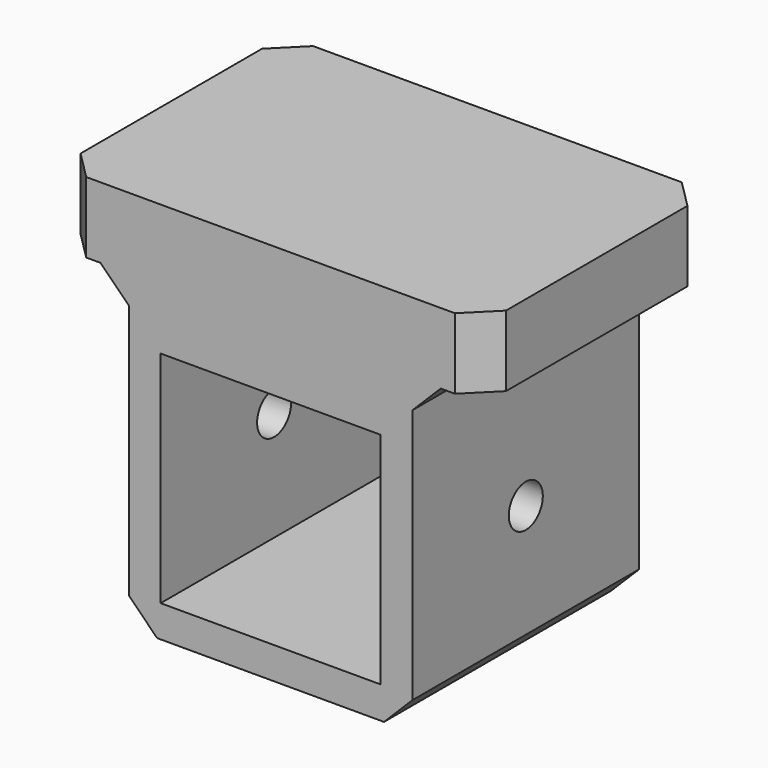
from build123d import *

# Parameters (mm, degrees)
F0_W          = 20
F0_H          = 22
F0_W_2        = 15.5
F0_H_2        = 15.5
F1_DEPTH      = 20
F2_SIZE       = 2
F3_R          = 1.5
F4_DEPTH      = 7.251
F4_DEPTH_BACK = 25


# Not quite as in the source:
# - a feature names something its author has since deleted; it is built from what else it names


with BuildPart() as f1:
    # F0 (on Front) → F1 (new body)
    with BuildSketch(Plane.XZ):
        with Locations((-38.0418774337, 18.7455339581)):
            Rectangle(F0_W, F0_H)
        with Locations((-38.0418774337, 17.7455339581)):
            Rectangle(F0_W_2, F0_H_2, mode=Mode.SUBTRACT)
        Polygon((-48.0418774337, 29.7455339581), (-28.0418774337, 29.7455339581), (-23.0418774337, 29.7455339581), (-23.0418774337, 34.7455339581), (-53.0418774337, 34.7455339581), (-53.0418774337, 29.7455339581), align=None)
    extrude(amount=F1_DEPTH)

    # F2
    f2_edges = [f1.edges().sort_by_distance(p)[0] for p in [
        (-28.041877, -10, 7.745534),
        (-48.041877, -10, 7.745534),
        (-48.041877, -10, 29.745534),
        (-28.041877, -10, 29.745534),
        (-23.041877, 0, 32.245534),
        (-53.041877, 0, 32.245534),
        (-53.041877, -20, 32.245534),
        (-23.041877, -20, 32.245534),
    ]]
    chamfer(f2_edges, length=F2_SIZE)

    # F3 (on face) → F4 (cut, two sides)
    with BuildSketch(Plane.YZ.offset(-45.7918774337)) as f4_sk:
        with Locations((-10, 17.7455339581)):
            Circle(F3_R)
    extrude(amount=-F4_DEPTH, mode=Mode.SUBTRACT)
    extrude(f4_sk.sketch, amount=F4_DEPTH_BACK, mode=Mode.SUBTRACT)


solid = f1.part
